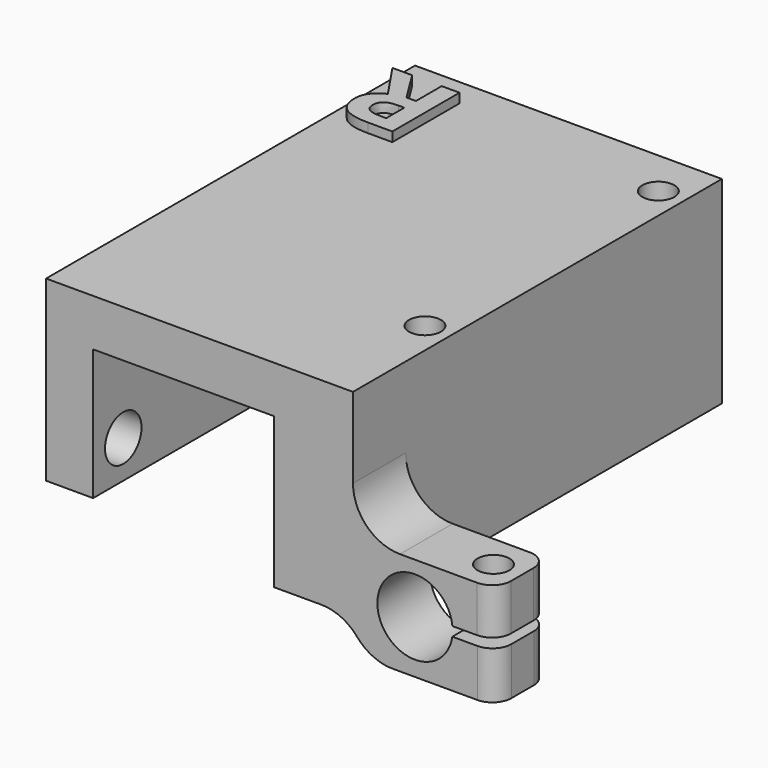
from build123d import *

# Parameters (mm, degrees)
F1_DEPTH      = 7
F2_DEPTH      = 42
F3_R          = 1.7
F3_R_2        = 11
F4_DEPTH      = 21.001
F5_R          = 4
F6_DEPTH      = 10
F7_DEPTH      = 21.001
F8_R          = 1.4
F9_DEPTH      = 11.0317641354
F8_R_2        = 1.7
F10_DEPTH     = 4.9110969969
F11_R         = 5
F12_R         = 5
F13_R         = 5
F14_R         = 2
F15_R         = 2.2
F15_R_2       = 2.4255023423
F16_DEPTH     = 6
F17_TEXT_SIZE = 12.5
F18_DEPTH     = 1


# Not quite as in the source:
# - a feature names something its author has since deleted; it is built from what else it names
# - Text() gives the source's letters only with a copy of the font that has no kerning and outlines rounded to 1/6400 em; it was checked with that copy


with BuildPart() as f1:
    # F0 (on Front) → F1 (new body)
    with BuildSketch(Plane.XZ):
        Polygon((-18.6721007523, 29.8099789735), (-18.6721007523, 10.8925135386), (-13.6721007523, 10.8925135386), (-13.6721007523, 24.8099789735), (5.5278992477, 24.8099789735), (5.5278992477, 8.8099789735), (13.9380548998, 8.8099789735), (13.9380548998, 16.2656020473), (13.9380548998, 29.8099789735), align=None)
        Polygon((29.1263195603, 16.2417280634), (13.9380548998, 16.2656020473), (13.9380548998, 8.8099789735), (15.3533044869, 5.2860832236), (29.1553367778, 5.2860832236), (29.1553367778, 10.343908232), (22.4860510706, 10.343908232), (22.4860510706, 11.3388913612), (29.1263195603, 11.3388913612), align=None)
    extrude(amount=F1_DEPTH)

    # F0 (on Front) → F2 (join)
    with BuildSketch(Plane.XZ):
        Polygon((-18.6721007523, 29.8099789735), (-18.6721007523, 10.8925135386), (-13.6721007523, 10.8925135386), (-13.6721007523, 24.8099789735), (5.5278992477, 24.8099789735), (5.5278992477, 8.8099789735), (13.9380548998, 8.8099789735), (13.9380548998, 16.2656020473), (13.9380548998, 29.8099789735), align=None)
    extrude(amount=-F2_DEPTH)

    # F3 (on face) → F4 (cut, through all)
    with BuildSketch(Plane(origin=(0, 0, 8.8099789735), x_dir=(1, 0, 0), z_dir=(0, 0, -1))):
        with Locations((11.1850741468, -6)):
            Circle(F3_R)
        with Locations((11.1850741468, -37)):
            Circle(F3_R)
        with Locations((26.6850741468, -21.5)):
            Circle(F3_R_2)
    extrude(amount=-F4_DEPTH, mode=Mode.SUBTRACT)

    # F5 (on face) → F6 (cut)
    with BuildSketch(Plane.XZ.offset(7)):
        with Locations((20.5278992477, 10.8989789735)):
            Circle(F5_R)
    extrude(amount=-F6_DEPTH, mode=Mode.SUBTRACT)

    # F3 (on face) → F7 (cut, through all)
    with BuildSketch(Plane(origin=(0, 0, 8.8099789735), x_dir=(1, 0, 0), z_dir=(0, 0, -1))):
        with Locations((11.1850741468, -6)):
            Circle(F3_R)
        with Locations((11.1850741468, -37)):
            Circle(F3_R)
        with Locations((26.6850741468, -21.5)):
            Circle(F3_R_2)
    extrude(amount=-F7_DEPTH, mode=Mode.SUBTRACT)

    # F8 (on face) → F9 (cut, through all)
    with BuildSketch(Plane(origin=(0.0256017933, 0, 16.2874706208), x_dir=(0.9999987646, 0, -0.0015718685), z_dir=(0.0015718685, 0, 0.9999987646))):
        with Locations((26.1007537177, -3.5767070949)):
            Circle(F8_R)
    extrude(amount=-F9_DEPTH, mode=Mode.SUBTRACT)

    # F8 (on face) → F10 (cut, through all)
    with BuildSketch(Plane(origin=(0.0256017933, 0, 16.2874706208), x_dir=(0.9999987646, 0, -0.0015718685), z_dir=(0.0015718685, 0, 0.9999987646))):
        with Locations((26.1007537177, -3.5767070949)):
            Circle(F8_R_2)
        with Locations((26.1007537177, -3.5767070949)):
            Circle(F8_R, mode=Mode.SUBTRACT)
    extrude(amount=-F10_DEPTH, mode=Mode.SUBTRACT)

    # F11
    f11_edges = [f1.edges().sort_by_distance(p)[0] for p in [
        (13.938055, -3.5, 16.265602),
    ]]
    fillet(f11_edges, radius=F11_R)

    # F12
    f12_edges = [f1.edges().sort_by_distance(p)[0] for p in [
        (13.938055, -3.5, 8.809979),
    ]]
    fillet(f12_edges, radius=F12_R)

    # F13
    f13_edges = [f1.edges().sort_by_distance(p)[0] for p in [
        (15.353304, -3.5, 5.286083),
    ]]
    fillet(f13_edges, radius=F13_R)

    # F14
    f14_edges = [f1.edges().sort_by_distance(p)[0] for p in [
        (29.12632, -7, 13.79031),
        (29.155337, -7, 7.814996),
        (29.12632, 0, 13.79031),
        (29.155337, 0, 7.814996),
    ]]
    fillet(f14_edges, radius=F14_R)

    # F15 (on face) → F16 (cut)
    with BuildSketch(Plane(origin=(-18.6721007523, 0, 0), x_dir=(0, -1, 0), z_dir=(-1, 0, 0))):
        with Locations((-38, 14.8925135386)):
            Circle(F15_R)
        with Locations((3, 14.8925135386)):
            Circle(F15_R_2)
    extrude(amount=-F16_DEPTH, mode=Mode.SUBTRACT)

    # F17 (on face) → F18 (join)
    with BuildSketch(Plane.XY.offset(29.8099789735)):
        with Locations(Location((-10.4201476273, 39), (0, 0, 180))):
            Text('R', F17_TEXT_SIZE, font='Open Sans', font_style=FontStyle.BOLD, text_align=(TextAlign.LEFT, TextAlign.BOTTOM))
    extrude(amount=F18_DEPTH)


solid = f1.part
